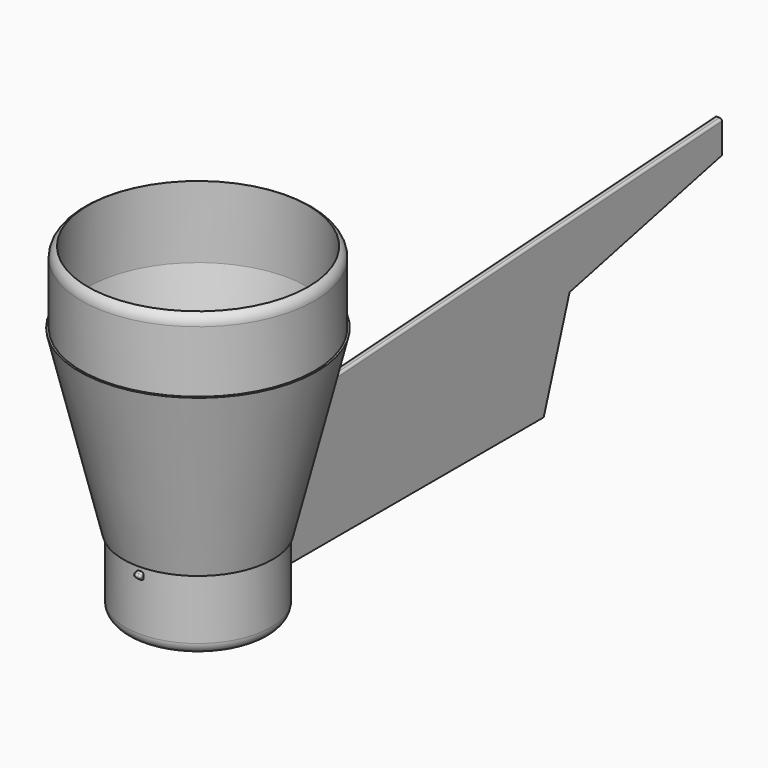
from build123d import *

# Parameters (mm, degrees)
F1_DEPTH     = 1
F2_R         = 0.625
F3_T1_DEPTH  = 65.0452526587
F3_T3_DEPTH  = 0.75
F3_T8_DEPTH  = 0.625
F3_T14_DEPTH = 0.625
F4_T1_DEPTH  = 28.8736358303
F4_T3_DEPTH  = 0.75
F4_T8_DEPTH  = 0.625
F4_T14_DEPTH = 0.625
F5_W         = 1.79999894
F5_H         = 20.0000108
F7_R         = 18.43110106
F8_DEPTH     = 2.00000108
F9_R         = 3.175


# Not quite as in the source:
# - a fillet or chamfer that OpenCascade refuses, or shapes differently, is made with other operations: its cross-section is extruded or revolved along the edge and cut away or added
# - a feature names something its author has since deleted; it is built from what else it names


with BuildPart() as f1:
    # F0 (on Right) → F1 (new body, symmetric)
    with BuildSketch(Plane.YZ):
        Polygon((-22, 18), (0, 0), (119, 0), (128, 27), (181, 39), (181, 48), (38, 39), align=None)
    extrude(amount=F1_DEPTH, both=True)

    # F2
    f2_edges = [f1.edges().sort_by_distance(p)[0] for p in [
        (1, 109.5, 43.5),
        (-1, 109.5, 43.5),
    ]]
    fillet(f2_edges, radius=F2_R)

    # F3: fillet of radius 0.625 on 2 edges, made by hand

    # F3_s2 → F3_t1 (cut)
    with BuildSketch(Plane(origin=(0, 45.932089611, 16.0762313638), x_dir=(1, 0, 0), z_dir=(0, -0.9438583564, -0.3303504247))):
        with BuildLine():
            ThreePointArc((-0.375, 24.2571597586), (-0.8169417382, 24.0741014968), (-1, 23.6321597586))
            Line((-1, 23.6321597586), (-1, 24.2571597586))
            Line((-1, 24.2571597586), (-0.375, 24.2571597586))
        make_face()
        with BuildLine():
            ThreePointArc((0.375, 24.2571597586), (0.8169417382, 24.0741014968), (1, 23.6321597586))
            Line((1, 23.6321597586), (1, 24.2571597586))
            Line((1, 24.2571597586), (0.375, 24.2571597586))
        make_face()
    extrude(amount=F3_T1_DEPTH, mode=Mode.SUBTRACT)

    # F3_s4 → F3_t3 (cut)
    with BuildSketch(Plane.YZ.offset(-0.375)):
        with BuildLine():
            ThreePointArc((37.918726582, 38.9715543037), (38.0011715289, 38.994213668), (38.0859376082, 39.0054086607))
            Line((38.0859376082, 39.0054086607), (38, 39))
            Line((38, 39), (37.918726582, 38.9715543037))
        make_face()
    extrude(amount=F3_T3_DEPTH, mode=Mode.SUBTRACT)


with BuildPart() as f3_tool6:
    # F3_s7 → F3_t8 (new body)
    with BuildSketch(Plane.YZ.offset(0.375)):
        Polygon((38.1251955975, 38.381642831), (37.918726582, 38.9715543037), (38, 39), (38.0859376082, 39.0054086607), align=None)
    extrude(amount=F3_T8_DEPTH)

    # F3_s9 → F3_t10 (revolve, cut)
    with BuildSketch(Plane(origin=(0.375, 38.1251955975, 38.381642831), x_dir=(0, 0.1984385097, -0.9801133393), z_dir=(0, -0.9801133393, -0.1984385097))):
        with BuildLine():
            ThreePointArc((0, -0.625), (0.625, 0), (0, 0.625))
            Line((0, 0.625), (0, -0.625))
        make_face()
    revolve(axis=Axis((0.375, 38.1251955975, 38.381642831), (1, 0, 0)), mode=Mode.SUBTRACT)


with BuildPart() as f1_1:
    add(f1.part)

    # F3_t5: cut F3_tool6
    add(f3_tool6.part, mode=Mode.SUBTRACT)


with BuildPart() as f3_tool12:
    # F3_s13 → F3_t14 (new body)
    with BuildSketch(Plane.YZ.offset(-0.375)):
        Polygon((38.1251955975, 38.381642831), (38.0859376082, 39.0054086607), (38, 39), (37.918726582, 38.9715543037), align=None)
    extrude(amount=-F3_T14_DEPTH)

    # F3_s15 → F3_t16 (revolve, cut)
    with BuildSketch(Plane(origin=(-0.375, 38.1251955975, 38.381642831), x_dir=(0, 0.1984385097, -0.9801133393), z_dir=(0, 0.9801133393, 0.1984385097))):
        with BuildLine():
            ThreePointArc((0, -0.625), (0.625, 0), (0, 0.625))
            Line((0, 0.625), (0, -0.625))
        make_face()
    revolve(axis=Axis((-0.375, 38.1251955975, 38.381642831), (-1, 0, 0)), mode=Mode.SUBTRACT)


with BuildPart() as f1_2:
    add(f1_1.part)

    # F3_t11: cut F3_tool12
    add(f3_tool12.part, mode=Mode.SUBTRACT)

    # F4: fillet of radius 0.625 on 3 edges, made by hand

    # F4_s2 → F4_t1 (cut)
    with BuildSketch(Plane(origin=(0, -21.1376529254, 17.2944433026), x_dir=(1, 0, 0), z_dir=(0, 0.7739572992, -0.6332377903))):
        with BuildLine():
            ThreePointArc((0.375, 0), (0.8169417382, -0.1830582618), (1, -0.625))
            Line((1, -0.625), (1, 0))
            Line((1, 0), (0.375, 0))
        make_face()
        with BuildLine():
            ThreePointArc((-0.375, 0), (-0.8169417382, -0.1830582618), (-1, -0.625))
            Line((-1, -0.625), (-1, 0))
            Line((-1, 0), (-0.375, 0))
        make_face()
    extrude(amount=F4_T1_DEPTH, mode=Mode.SUBTRACT)

    # F4_s4 → F4_t3 (cut)
    with BuildSketch(Plane.YZ.offset(-0.375)):
        with BuildLine():
            ThreePointArc((-20.9483483219, 18.3680780873), (-21.3573847576, 17.8866932915), (-21.1376529254, 17.2944433026))
            Line((-21.1376529254, 17.2944433026), (-22, 18))
            Line((-22, 18), (-20.9483483219, 18.3680780873))
        make_face()
    extrude(amount=F4_T3_DEPTH, mode=Mode.SUBTRACT)


with BuildPart() as f4_tool6:
    # F4_s7 → F4_t8 (new body)
    with BuildSketch(Plane.YZ.offset(0.375)):
        Polygon((-20.7418793065, 17.7781666146), (-21.1376529254, 17.2944433026), (-22, 18), (-20.9483483219, 18.3680780873), align=None)
    extrude(amount=F4_T8_DEPTH)

    # F4_s9 → F4_t10 (revolve, cut)
    with BuildSketch(Plane(origin=(0.375, -20.7418793065, 17.7781666146), x_dir=(0, 0.9848087219, -0.173642683), z_dir=(0, -0.173642683, -0.9848087219))):
        with BuildLine():
            ThreePointArc((0, -0.625), (0.625, 0), (0, 0.625))
            Line((0, 0.625), (0, -0.625))
        make_face()
    revolve(axis=Axis((0.375, -20.7418793065, 17.7781666146), (1, 0, 0)), mode=Mode.SUBTRACT)


with BuildPart() as f1_3:
    add(f1_2.part)

    # F4_t5: cut F4_tool6
    add(f4_tool6.part, mode=Mode.SUBTRACT)


with BuildPart() as f4_tool12:
    # F4_s13 → F4_t14 (new body)
    with BuildSketch(Plane.YZ.offset(-0.375)):
        Polygon((-20.7418793065, 17.7781666146), (-21.1376529254, 17.2944433026), (-22, 18), (-20.9483483219, 18.3680780873), align=None)
    extrude(amount=-F4_T14_DEPTH)

    # F4_s15 → F4_t16 (revolve, cut)
    with BuildSketch(Plane(origin=(-0.375, -20.7418793065, 17.7781666146), x_dir=(0, 0.9848087219, -0.173642683), z_dir=(0, 0.173642683, 0.9848087219))):
        with BuildLine():
            ThreePointArc((0, -0.625), (0.625, 0), (0, 0.625))
            Line((0, 0.625), (0, -0.625))
        make_face()
    revolve(axis=Axis((-0.375, -20.7418793065, 17.7781666146), (-1, 0, 0)), mode=Mode.SUBTRACT)


with BuildPart() as f1_4:
    add(f1_3.part)

    # F4_t11: cut F4_tool12
    add(f4_tool12.part, mode=Mode.SUBTRACT)


with BuildPart() as f6:
    # F5 (on Front) → F6 (revolve)
    with BuildSketch(Plane.XZ):
        Polygon((32.4739, 69.9999108), (30.67390106, 69.9999108), (18.43110106, 20.0000108), (20.2311, 20.0000108), (20.7899, 20.0000108), (33.02, 69.9999108), align=None)
        with Locations((19.33110053, 10.0000054)):
            Rectangle(F5_W, F5_H)
        with Locations((31.57390053, 79.9999162)):
            Rectangle(F5_W, F5_H)
    revolve(axis=Axis((0, 0, -0.9119894143), (0, 0, -1)))

    # F7 (on Top) → F8 (join)
    with BuildSketch(Plane.XY):
        Circle(F7_R)
    extrude(amount=F8_DEPTH)

    # F9
    f9_edges = [f6.edges().sort_by_distance(p)[0] for p in [
        (-20.2311, 0, 0),
    ]]
    fillet(f9_edges, radius=F9_R)

    # F10: fillet of radius 3.175 on 1 edges, made by hand

    # F10_s1 → F10_t2 (revolve, cut)
    with BuildSketch(Plane.XZ):
        with BuildLine():
            ThreePointArc((32.4739, 87.138104505), (31.9864875209, 88.8285181577), (30.67390106, 89.9999216))
            Line((30.67390106, 89.9999216), (32.4739, 89.9999216))
            Line((32.4739, 89.9999216), (32.4739, 87.138104505))
        make_face()
    revolve(axis=Axis((0, 0, 89.9999216), (0, 0, -1)), mode=Mode.SUBTRACT)


solid = Compound([f1_4.part, f6.part])
